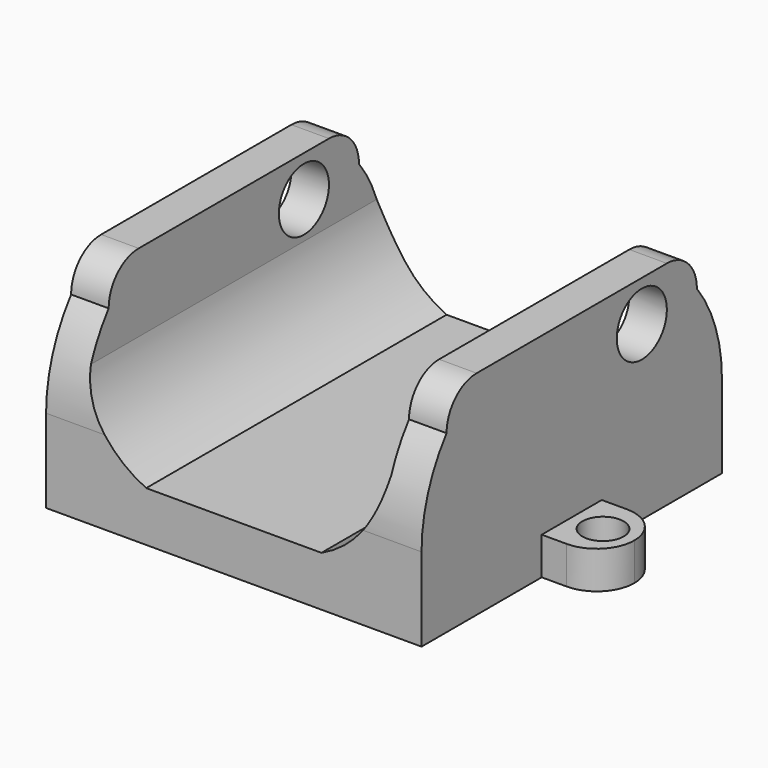
from build123d import *

# Parameters (mm, degrees)
F0_W         = 30
F0_H         = 30
F1_DEPTH     = 4
F2_W         = 3
F2_H         = 10
F3_DEPTH     = 15
F5_DEPTH     = 15
F6_W         = 5
F6_H         = 3
F7_DEPTH     = 3
F8_R         = 2.99999
F9_R         = 1.65
F10_DEPTH    = 25
F11_W        = 3
F11_H        = 3
F12_DEPTH    = 12.5
F13_R        = 2.99999
F14_R        = 2.5
F15_DEPTH    = 18.8
F16_T1_DEPTH = 39.6571957465
F16_T3_DEPTH = 39.6571957465


# Not quite as in the source:
# - a fillet or chamfer that OpenCascade refuses, or shapes differently, is made with other operations: its cross-section is extruded or revolved along the edge and cut away or added
# - a fillet or chamfer is up to 0.001 mm smaller than in the source, because OpenCascade refuses the exact size


with BuildPart() as f1:
    # F0 (on Top) → F1 (new body)
    with BuildSketch(Plane.XY):
        Rectangle(F0_W, F0_H)
    extrude(amount=-F1_DEPTH)

    # F2 (on Front) → F3 (join, symmetric)
    with BuildSketch(Plane.XZ):
        with Locations((-13.5, 5)):
            Rectangle(F2_W, F2_H)
        with Locations((13.5, 5)):
            Rectangle(F2_W, F2_H)
    extrude(amount=F3_DEPTH, both=True)

    # F4 (on Front) → F5 (join, symmetric)
    with BuildSketch(Plane.XZ):
        with BuildLine():
            Line((-12, 6.7849478247), (-12, 9))
            ThreePointArc((-12, 9), (-12.0709686948, 7.8924739124), (-12, 6.7849478247))
        make_face()
        with BuildLine():
            ThreePointArc((-7, 0), (-10.3790782907, 2.7446588419), (-12, 6.7849478247))
            Line((-12, 6.7849478247), (-12, 0))
            Line((-12, 0), (-7, 0))
        make_face()
        with BuildLine():
            Line((12, 0), (12, 6.7849478247))
            ThreePointArc((12, 6.7849478247), (10.3790782907, 2.7446588419), (7, 0))
            Line((7, 0), (12, 0))
        make_face()
        with BuildLine():
            ThreePointArc((12, 6.7849478247), (12.0709686948, 7.8924739124), (12, 9))
            Line((12, 9), (12, 6.7849478247))
        make_face()
    extrude(amount=F5_DEPTH, both=True)

    # F6 (on Front) → F7 (join, symmetric)
    with BuildSketch(Plane.XZ):
        with Locations((-17.5, -2.5)):
            Rectangle(F6_W, F6_H)
        with Locations((17.5, -2.5)):
            Rectangle(F6_W, F6_H)
    extrude(amount=F7_DEPTH, both=True)

    # F8 (radius 3 in the source; OpenCascade refuses exactly that, so slightly less here)
    f8_edges = [f1.edges().sort_by_distance(p)[0] for p in [
        (-20, 3, -2.5),
        (-20, -3, -2.5),
        (20, 3, -2.5),
        (20, -3, -2.5),
    ]]
    fillet(f8_edges, radius=F8_R)

    # F9 (on Top) → F10 (cut)
    with BuildSketch(Plane.XY):
        with Locations((-17.5, 0)):
            Circle(F9_R)
        with Locations((17.5, 0)):
            Circle(F9_R)
    extrude(amount=-F10_DEPTH, mode=Mode.SUBTRACT)

    # F11 (on Front) → F12 (join, symmetric)
    with BuildSketch(Plane.XZ):
        with Locations((-13.5, 11.5)):
            Rectangle(F11_W, F11_H)
        with Locations((13.5, 11.5)):
            Rectangle(F11_W, F11_H)
    extrude(amount=F12_DEPTH, both=True)

    # F13 (radius 3 in the source; OpenCascade refuses exactly that, so slightly less here)
    f13_edges = [f1.edges().sort_by_distance(p)[0] for p in [
        (-13.5, -12.5, 13),
        (-13.5, 12.5, 13),
        (13.5, -12.5, 13),
        (13.5, 12.5, 13),
    ]]
    fillet(f13_edges, radius=F13_R)

    # F14 (on Right) → F15 (cut, symmetric)
    with BuildSketch(Plane.YZ):
        with Locations((7, 9.75)):
            Circle(F14_R)
    extrude(amount=F15_DEPTH, both=True, mode=Mode.SUBTRACT)

    # F16: fillet of radius 12 on 4 edges, made by hand

    # F16_s2 → F16_t1 (cut)
    with BuildSketch(Plane.YZ.offset(-6.3285978733)):
        with BuildLine():
            ThreePointArc((15, 2.6685608507), (14.3578166916, 6.5415441969), (12.5, 10))
            Line((12.5, 10), (15, 10))
            Line((15, 10), (15, 2.6685608507))
        make_face()
        with BuildLine():
            ThreePointArc((-15, 2.6685608507), (-14.3578166916, 6.5415441969), (-12.5, 10))
            Line((-12.5, 10), (-15, 10))
            Line((-15, 10), (-15, 2.6685608507))
        make_face()
    extrude(amount=F16_T1_DEPTH, mode=Mode.SUBTRACT)

    # F16_s4 → F16_t3 (cut)
    with BuildSketch(Plane.YZ.offset(-33.3285978733)):
        with BuildLine():
            ThreePointArc((-12.5, 10), (-14.3578166916, 6.5415441969), (-15, 2.6685608507))
            Line((-15, 2.6685608507), (-15, 10))
            Line((-15, 10), (-12.5, 10))
        make_face()
        with BuildLine():
            ThreePointArc((12.5, 10), (14.3578166916, 6.5415441969), (15, 2.6685608507))
            Line((15, 2.6685608507), (15, 10))
            Line((15, 10), (12.5, 10))
        make_face()
    extrude(amount=F16_T3_DEPTH, mode=Mode.SUBTRACT)


solid = f1.part
